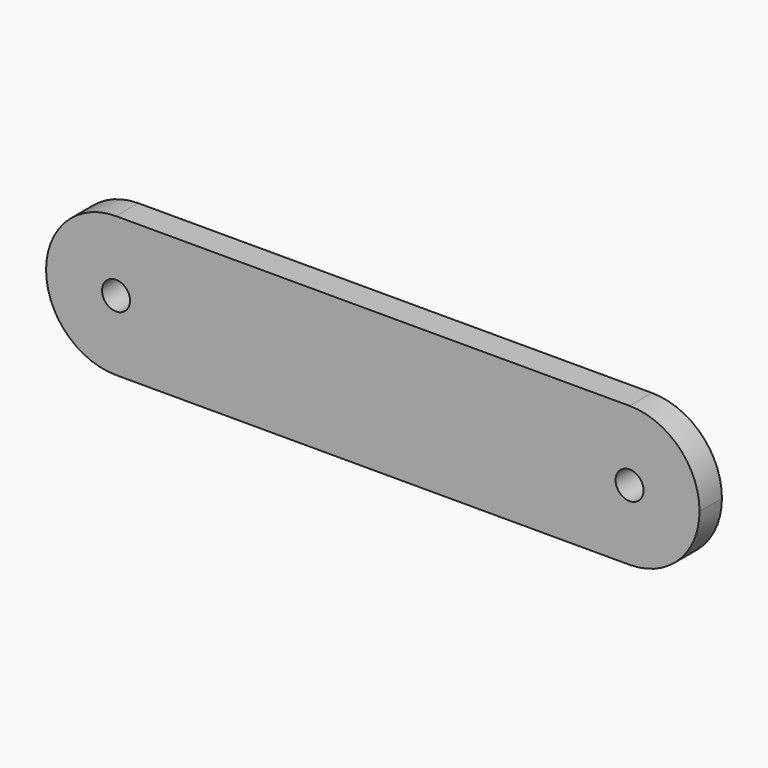
from build123d import *

# Parameters (mm, degrees)
F0_W     = 46.7
F0_H     = 10
F0_R     = 1
F1_DEPTH = 2
F2_R     = 4.99999


# Not quite as in the source:
# - a fillet or chamfer is up to 0.001 mm smaller than in the source, because OpenCascade refuses the exact size


with BuildPart() as f1:
    # F0 (on Front) → F1 (new body)
    with BuildSketch(Plane.XZ):
        with Locations((23.35, -5)):
            Rectangle(F0_W, F0_H)
        with Locations((5, -5)):
            Circle(F0_R, mode=Mode.SUBTRACT)
        with Locations((41.7, -5)):
            Circle(F0_R, mode=Mode.SUBTRACT)
    extrude(amount=F1_DEPTH)

    # F2 (radius 5 in the source; OpenCascade refuses exactly that, so slightly less here)
    f2_edges = [f1.edges().sort_by_distance(p)[0] for p in [
        (0, -1, 0),
        (0, -1, -10),
        (46.7, -1, 0),
        (46.7, -1, -10),
    ]]
    fillet(f2_edges, radius=F2_R)


solid = f1.part
